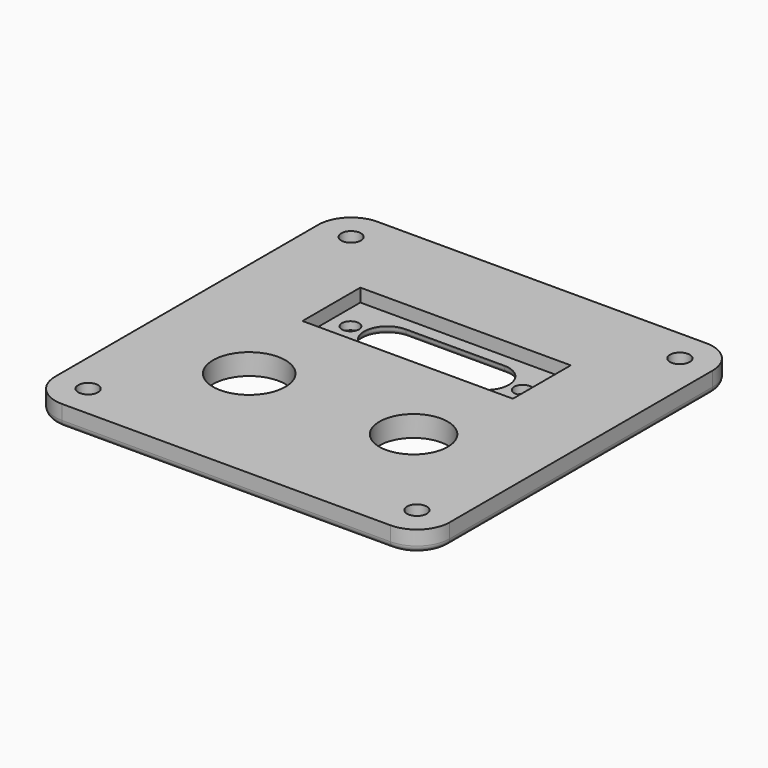
from build123d import *

# Parameters (mm, degrees)
F0_W         = 76.2
F0_H         = 76.2
F0_R         = 1.905
F0_R_2       = 6.985
F0_R_3       = 6.604
F0_R_4       = 1.651
F1_DEPTH     = 1.524
F2_W         = 76.2
F2_H         = 76.2
F2_R         = 1.905
F2_W_2       = 40.64
F2_H_2       = 13.97
F3_DEPTH     = 2.54
F4_R         = 6.35
F5_T1_DEPTH  = 19.05
F5_T3_DEPTH  = 63.5
F5_T5_DEPTH  = 63.5
F5_T8_ANGLE  = 90
F5_T10_ANGLE = 90
F5_T12_ANGLE = 90
F5_T14_ANGLE = 90
F5_T16_ANGLE = 180
F5_T18_ANGLE = 180
F6_DEPTH     = 2.54


# Not quite as in the source:
# - a fillet or chamfer that OpenCascade refuses, or shapes differently, is made with other operations: its cross-section is extruded or revolved along the edge and cut away or added
# - a feature names something its author has since deleted; it is built from what else it names


with BuildPart() as f1:
    # F0 (on Top) → F1 (new body)
    with BuildSketch(Plane.XY):
        with Locations((0, -12.7)):
            Rectangle(F0_W, F0_H)
        with Locations((-31.75, -44.45)):
            Circle(F0_R, mode=Mode.SUBTRACT)
        with Locations((-15.875, -25.4)):
            Circle(F0_R_2, mode=Mode.SUBTRACT)
        with Locations((31.75, -44.45)):
            Circle(F0_R, mode=Mode.SUBTRACT)
        with Locations((15.875, -25.4)):
            Circle(F0_R_3, mode=Mode.SUBTRACT)
        with Locations((-16.637, 0)):
            Circle(F0_R_4, mode=Mode.SUBTRACT)
        with Locations((-31.75, 19.05)):
            Circle(F0_R, mode=Mode.SUBTRACT)
        with BuildLine():
            ThreePointArc((-9.525, -4.445), (-13.97, 0), (-9.525, 4.445))
            Line((-9.525, 4.445), (9.525, 4.445))
            ThreePointArc((9.525, 4.445), (13.97, 0), (9.525, -4.445))
            Line((9.525, -4.445), (-9.525, -4.445))
        make_face(mode=Mode.SUBTRACT)
        with Locations((16.637, 0)):
            Circle(F0_R_4, mode=Mode.SUBTRACT)
        with Locations((31.75, 19.05)):
            Circle(F0_R, mode=Mode.SUBTRACT)
    extrude(amount=F1_DEPTH)

    # F2 (on face) → F3 (join)
    with BuildSketch(Plane.XY.offset(1.524)):
        with Locations((0, -12.7)):
            Rectangle(F2_W, F2_H)
        with Locations((-31.75, -44.45)):
            Circle(F2_R, mode=Mode.SUBTRACT)
        with Locations((31.75, -44.45)):
            Circle(F2_R, mode=Mode.SUBTRACT)
        with Locations((-31.75, 19.05)):
            Circle(F2_R, mode=Mode.SUBTRACT)
        Rectangle(F2_W_2, F2_H_2, mode=Mode.SUBTRACT)
        with Locations((31.75, 19.05)):
            Circle(F2_R, mode=Mode.SUBTRACT)
    extrude(amount=F3_DEPTH)

    # F4
    f4_edges = [f1.edges().sort_by_distance(p)[0] for p in [
        (-38.1, -50.8, 2.032),
        (38.1, -50.8, 2.032),
        (-38.1, 25.4, 2.032),
        (38.1, 25.4, 2.032),
    ]]
    fillet(f4_edges, radius=F4_R)

    # F5: fillet of radius 1.27 on 12 edges, made by hand

    # F5_s2 → F5_t1 (cut)
    with BuildSketch(Plane.YZ.offset(-9.525)):
        with BuildLine():
            ThreePointArc((5.715, 0), (4.8169743879, 0.3719743879), (4.445, 1.27))
            Line((4.445, 1.27), (4.445, 0))
            Line((4.445, 0), (5.715, 0))
        make_face()
        with BuildLine():
            ThreePointArc((-5.715, 0), (-4.8169743879, 0.3719743879), (-4.445, 1.27))
            Line((-4.445, 1.27), (-4.445, 0))
            Line((-4.445, 0), (-5.715, 0))
        make_face()
    extrude(amount=F5_T1_DEPTH, mode=Mode.SUBTRACT)

    # F5_s4 → F5_t3 (cut)
    with BuildSketch(Plane.XZ.offset(-19.05)):
        with BuildLine():
            ThreePointArc((38.1, 1.27), (37.7280256121, 0.3719743879), (36.83, 0))
            Line((36.83, 0), (38.1, 0))
            Line((38.1, 0), (38.1, 1.27))
        make_face()
        with BuildLine():
            ThreePointArc((-36.83, 0), (-37.7280256121, 0.3719743879), (-38.1, 1.27))
            Line((-38.1, 1.27), (-38.1, 0))
            Line((-38.1, 0), (-36.83, 0))
        make_face()
    extrude(amount=F5_T3_DEPTH, mode=Mode.SUBTRACT)

    # F5_s6 → F5_t5 (cut)
    with BuildSketch(Plane.YZ.offset(-31.75)):
        with BuildLine():
            ThreePointArc((-49.53, 0), (-50.4280256121, 0.3719743879), (-50.8, 1.27))
            Line((-50.8, 1.27), (-50.8, 0))
            Line((-50.8, 0), (-49.53, 0))
        make_face()
        with BuildLine():
            ThreePointArc((24.13, 0), (25.0280256121, 0.3719743879), (25.4, 1.27))
            Line((25.4, 1.27), (25.4, 0))
            Line((25.4, 0), (24.13, 0))
        make_face()
    extrude(amount=F5_T5_DEPTH, mode=Mode.SUBTRACT)

    # F5_s7 → F5_t8 (revolve, cut)
    with BuildSketch(Plane.XZ.offset(44.45)):
        with BuildLine():
            ThreePointArc((-36.83, 0), (-37.7280256121, 0.3719743879), (-38.1, 1.27))
            Line((-38.1, 1.27), (-38.1, 0))
            Line((-38.1, 0), (-36.83, 0))
        make_face()
    revolve(axis=Axis((-31.75, -44.45, 0), (0, 0, 1)), revolution_arc=F5_T8_ANGLE, mode=Mode.SUBTRACT)

    # F5_s9 → F5_t10 (revolve, cut)
    with BuildSketch(Plane.XZ.offset(44.45)):
        with BuildLine():
            ThreePointArc((38.1, 1.27), (37.7280256121, 0.3719743879), (36.83, 0))
            Line((36.83, 0), (38.1, 0))
            Line((38.1, 0), (38.1, 1.27))
        make_face()
    revolve(axis=Axis((31.75, -44.45, 0), (0, 0, -1)), revolution_arc=F5_T10_ANGLE, mode=Mode.SUBTRACT)

    # F5_s11 → F5_t12 (revolve, cut)
    with BuildSketch(Plane.XZ.offset(-19.05)):
        with BuildLine():
            ThreePointArc((38.1, 1.27), (37.7280256121, 0.3719743879), (36.83, 0))
            Line((36.83, 0), (38.1, 0))
            Line((38.1, 0), (38.1, 1.27))
        make_face()
    revolve(axis=Axis((31.75, 19.05, 0), (0, 0, 1)), revolution_arc=F5_T12_ANGLE, mode=Mode.SUBTRACT)

    # F5_s13 → F5_t14 (revolve, cut)
    with BuildSketch(Plane.XZ.offset(-19.05)):
        with BuildLine():
            ThreePointArc((-36.83, 0), (-37.7280256121, 0.3719743879), (-38.1, 1.27))
            Line((-38.1, 1.27), (-38.1, 0))
            Line((-38.1, 0), (-36.83, 0))
        make_face()
    revolve(axis=Axis((-31.75, 19.05, 0), (0, 0, -1)), revolution_arc=F5_T14_ANGLE, mode=Mode.SUBTRACT)

    # F5_s15 → F5_t16 (revolve, cut)
    with BuildSketch(Plane.YZ.offset(-9.525)):
        with BuildLine():
            ThreePointArc((-5.715, 0), (-4.8169743879, 0.3719743879), (-4.445, 1.27))
            Line((-4.445, 1.27), (-4.445, 0))
            Line((-4.445, 0), (-5.715, 0))
        make_face()
    revolve(axis=Axis((-9.525, 0, 0), (0, 0, -1)), revolution_arc=F5_T16_ANGLE, mode=Mode.SUBTRACT)

    # F5_s17 → F5_t18 (revolve, cut)
    with BuildSketch(Plane.YZ.offset(9.525)):
        with BuildLine():
            ThreePointArc((5.715, 0), (4.8169743879, 0.3719743879), (4.445, 1.27))
            Line((4.445, 1.27), (4.445, 0))
            Line((4.445, 0), (5.715, 0))
        make_face()
    revolve(axis=Axis((9.525, 0, 0), (0, 0, -1)), revolution_arc=F5_T18_ANGLE, mode=Mode.SUBTRACT)

    # F6 (cut, through all): faces of the model
    f6_faces = [f1.faces().sort_by_distance(p)[0] for p in [
        (15.875, -25.4, 1.524),
        (-15.875, -25.4, 1.524),
    ]]
    extrude(f6_faces, amount=-F6_DEPTH, mode=Mode.SUBTRACT)


solid = f1.part
